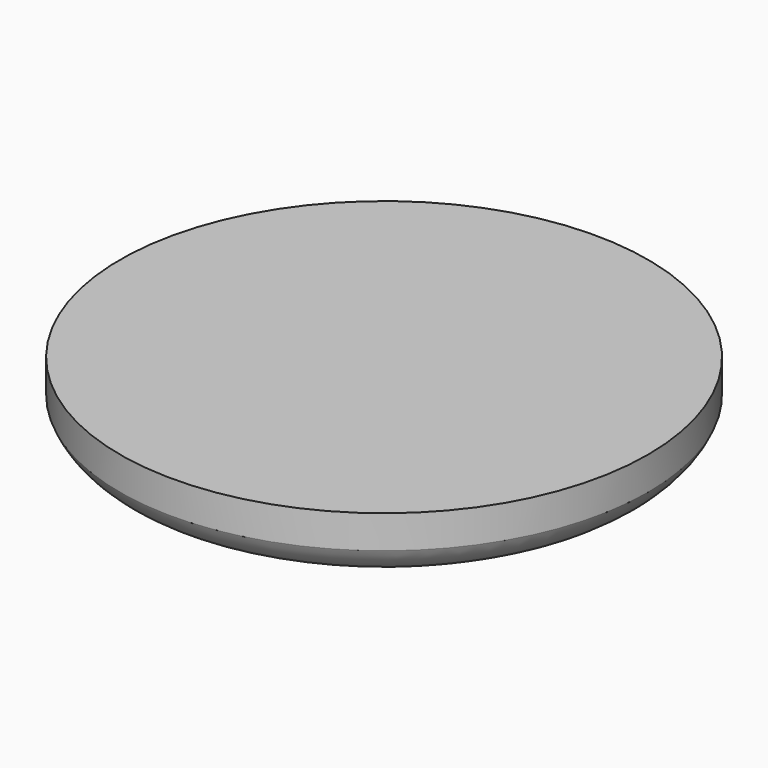
from build123d import *

# Parameters (mm, degrees)
F0_R     = 2.3
F1_DEPTH = 1.25
F0_R_2   = 10
F3_START = 1.25
F3_DEPTH = 1.25


# Not quite as in the source:
# - a fillet or chamfer that OpenCascade refuses, or shapes differently, is made with other operations: its cross-section is extruded or revolved along the edge and cut away or added


with BuildPart() as f1:
    # F0 (on Top) → F1 (new body)
    with BuildSketch(Plane.XY):
        Circle(F0_R)
    extrude(amount=F1_DEPTH)


with BuildPart() as f1b:
    # F0 (on Top) → F1, piece 2 (new body)
    with BuildSketch(Plane.XY):
        Circle(F0_R_2)
        with BuildLine():
            ThreePointArc((2.1072346154, -8.7498321284), (-2.5499973556, -8.6311942098), (-6.5239595944, -6.1998347729))
            Line((-6.5239595944, -6.1998347729), (-2.3921185179, -2.27327275))
            ThreePointArc((-2.3921185179, -2.27327275), (-3.2082717804, -0.7726526923), (-3.1647712102, 0.9349990304))
            Line((-3.1647712102, 0.9349990304), (-8.6311942098, 2.5499973556))
            ThreePointArc((-8.6311942098, 2.5499973556), (-6.1998347729, 6.5239595944), (-2.1072346154, 8.7498321284))
            Line((-2.1072346154, 8.7498321284), (-0.7726526923, 3.2082717804))
            ThreePointArc((-0.7726526923, 3.2082717804), (0.9349990304, 3.1647712102), (2.3921185179, 2.27327275))
            Line((2.3921185179, 2.27327275), (6.5239595944, 6.1998347729))
            ThreePointArc((6.5239595944, 6.1998347729), (8.7498321284, 2.1072346154), (8.6311942098, -2.5499973556))
            Line((8.6311942098, -2.5499973556), (3.1647712102, -0.9349990304))
            ThreePointArc((3.1647712102, -0.9349990304), (2.27327275, -2.3921185179), (0.7726526923, -3.2082717804))
            Line((0.7726526923, -3.2082717804), (2.1072346154, -8.7498321284))
        make_face(mode=Mode.SUBTRACT)
    extrude(amount=F1_DEPTH)

    # F2: fillet of radius 2 on 1 edges, made by hand

    # F2_s1 → F2_t2 (revolve, cut)
    with BuildSketch(Plane.XZ):
        with BuildLine():
            ThreePointArc((10, 1.25), (9.263984367, 0.3416876048), (8.1459503782, 0))
            Line((8.1459503782, 0), (10, 0))
            Line((10, 0), (10, 1.25))
        make_face()
    revolve(axis=Axis((0, 0, 0), (0, 0, 1)), mode=Mode.SUBTRACT)


with BuildPart() as f3:
    # F0 (on Top) → F3 (new body)
    with BuildSketch(Plane.XY.offset(F3_START)):
        Circle(F0_R_2)
        with BuildLine():
            ThreePointArc((2.1072346154, -8.7498321284), (-2.5499973556, -8.6311942098), (-6.5239595944, -6.1998347729))
            Line((-6.5239595944, -6.1998347729), (-2.3921185179, -2.27327275))
            ThreePointArc((-2.3921185179, -2.27327275), (-3.2082717804, -0.7726526923), (-3.1647712102, 0.9349990304))
            Line((-3.1647712102, 0.9349990304), (-8.6311942098, 2.5499973556))
            ThreePointArc((-8.6311942098, 2.5499973556), (-6.1998347729, 6.5239595944), (-2.1072346154, 8.7498321284))
            Line((-2.1072346154, 8.7498321284), (-0.7726526923, 3.2082717804))
            ThreePointArc((-0.7726526923, 3.2082717804), (0.9349990304, 3.1647712102), (2.3921185179, 2.27327275))
            Line((2.3921185179, 2.27327275), (6.5239595944, 6.1998347729))
            ThreePointArc((6.5239595944, 6.1998347729), (8.7498321284, 2.1072346154), (8.6311942098, -2.5499973556))
            Line((8.6311942098, -2.5499973556), (3.1647712102, -0.9349990304))
            ThreePointArc((3.1647712102, -0.9349990304), (2.27327275, -2.3921185179), (0.7726526923, -3.2082717804))
            Line((0.7726526923, -3.2082717804), (2.1072346154, -8.7498321284))
        make_face(mode=Mode.SUBTRACT)
        with BuildLine():
            Line((-2.3921185179, -2.27327275), (-6.5239595944, -6.1998347729))
            ThreePointArc((-6.5239595944, -6.1998347729), (-2.5499973556, -8.6311942098), (2.1072346154, -8.7498321284))
            Line((2.1072346154, -8.7498321284), (0.7726526923, -3.2082717804))
            ThreePointArc((0.7726526923, -3.2082717804), (2.27327275, -2.3921185179), (3.1647712102, -0.9349990304))
            Line((3.1647712102, -0.9349990304), (8.6311942098, -2.5499973556))
            ThreePointArc((8.6311942098, -2.5499973556), (8.7498321284, 2.1072346154), (6.5239595944, 6.1998347729))
            Line((6.5239595944, 6.1998347729), (2.3921185179, 2.27327275))
            ThreePointArc((2.3921185179, 2.27327275), (0.9349990304, 3.1647712102), (-0.7726526923, 3.2082717804))
            Line((-0.7726526923, 3.2082717804), (-2.1072346154, 8.7498321284))
            ThreePointArc((-2.1072346154, 8.7498321284), (-6.1998347729, 6.5239595944), (-8.6311942098, 2.5499973556))
            Line((-8.6311942098, 2.5499973556), (-3.1647712102, 0.9349990304))
            ThreePointArc((-3.1647712102, 0.9349990304), (-3.2082717804, -0.7726526923), (-2.3921185179, -2.27327275))
        make_face()
        Circle(F0_R, mode=Mode.SUBTRACT)
        Circle(F0_R)
    extrude(amount=F3_DEPTH)


solid = Compound([f1.part, f1b.part, f3.part])
